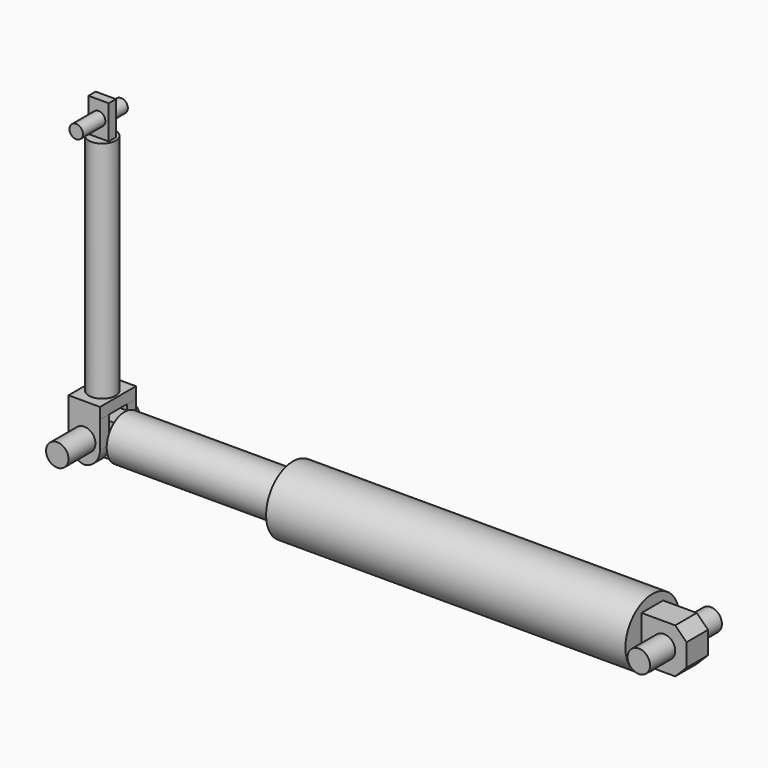
from build123d import *

# Parameters (mm, degrees)
F0_R         = 10
F1_DEPTH     = 75
F2_R         = 15
F2_R_2       = 10
F3_DEPTH     = 150
F4_R         = 15
F5_DEPTH     = 10
F6_W         = 12
F6_H         = 20
F7_DEPTH     = 20
F8_R         = 5
F9_DEPTH     = 21.001
F10_SIZE     = 5
F11_W        = 10
F11_H        = 15
F12_DEPTH    = 20
F13_R        = 5
F14_DEPTH    = 20.001
F15_R        = 5
F16_DEPTH    = 20
F17_W        = 14
F17_H        = 5
F18_DEPTH    = 10
F19_W        = 14.032341361
F19_H        = 20.0174024701
F20_DEPTH    = 5
F21_R        = 5
F22_DEPTH    = 20
F24_T1_DEPTH = 45
F24_T3_DEPTH = 45
F25_R        = 6
F26_DEPTH    = 100
F27_W        = 9
F27_H        = 4
F28_DEPTH    = 15
F29_R        = 3
F30_DEPTH    = 12.5
F32_T1_DEPTH = 50


# Not quite as in the source:
# - a fillet or chamfer that OpenCascade refuses, or shapes differently, is made with other operations: its cross-section is extruded or revolved along the edge and cut away or added


with BuildPart() as f1:
    # F0 (on Right) → F1 (new body, symmetric)
    with BuildSketch(Plane.YZ):
        Circle(F0_R)
    extrude(amount=F1_DEPTH, both=True)

    # F11 (on face) → F12 (join)
    with BuildSketch(Plane(origin=(-75, 0, 0), x_dir=(0, -1, 0), z_dir=(-1, 0, 0))):
        Rectangle(F11_W, F11_H)
    extrude(amount=F12_DEPTH)

    # F13 (on face) → F14 (cut, through all)
    with BuildSketch(Plane.XZ.offset(5)):
        with Locations((-85, 0)):
            Circle(F13_R)
    extrude(amount=-F14_DEPTH, mode=Mode.SUBTRACT)

    # F32: fillet of radius 8 on 2 edges, made by hand

    # F32_s2 → F32_t1 (cut)
    with BuildSketch(Plane.XZ.offset(-25)):
        with BuildLine():
            ThreePointArc((-87, 7.5), (-92.6568542495, 5.1568542495), (-95, -0.5))
            Line((-95, -0.5), (-95, 7.5))
            Line((-95, 7.5), (-87, 7.5))
        make_face()
        with BuildLine():
            ThreePointArc((-87, -7.5), (-92.6568542495, -5.1568542495), (-95, 0.5))
            Line((-95, 0.5), (-95, -7.5))
            Line((-95, -7.5), (-87, -7.5))
        make_face()
    extrude(amount=F32_T1_DEPTH, mode=Mode.SUBTRACT)


with BuildPart() as f3:
    # F2 (on Right) → F3 (new body)
    with BuildSketch(Plane.YZ):
        Circle(F2_R)
        Circle(F2_R_2, mode=Mode.SUBTRACT)
    extrude(amount=F3_DEPTH)

    # F4 (on face) → F5 (join)
    with BuildSketch(Plane.YZ.offset(150)):
        Circle(F4_R)
    extrude(amount=F5_DEPTH)

    # F6 (on face) → F7 (join)
    with BuildSketch(Plane.YZ.offset(160)):
        Rectangle(F6_W, F6_H)
    extrude(amount=F7_DEPTH)

    # F8 (on face) → F9 (cut, through all)
    with BuildSketch(Plane.XZ.offset(6)):
        with Locations((170, 0)):
            Circle(F8_R)
    extrude(amount=-F9_DEPTH, mode=Mode.SUBTRACT)

    # F10
    f10_edges = [f3.edges().sort_by_distance(p)[0] for p in [
        (180, 0, 10),
        (180, 0, -10),
    ]]
    chamfer(f10_edges, length=F10_SIZE)


with BuildPart() as f16:
    # F15 (on Front) → F16 (new body, symmetric)
    with BuildSketch(Plane.XZ):
        with Locations((170, 0)):
            Circle(F15_R)
    extrude(amount=F16_DEPTH, both=True)


with BuildPart() as f18:
    # F17 (on Top) → F18 (new body, symmetric)
    with BuildSketch(Plane.XY):
        with Locations((-85, 7.5)):
            Rectangle(F17_W, F17_H)
    extrude(amount=F18_DEPTH, both=True)



with BuildPart() as f18b:
    # F17 (on Top) → F18, piece 2 (new body, symmetric)
    with BuildSketch(Plane.XY):
        with Locations((-85, -7.5)):
            Rectangle(F17_W, F17_H)
    extrude(amount=F18_DEPTH, both=True)


with BuildPart() as f18_1:
    add(f18.part)

    add(f18b.part)  # F20 merges F18b
    # F19 (on face) → F20 (join)
    with BuildSketch(Plane.XY.offset(10)):
        with Locations((-84.9838293195, 0.0087012351)):
            Rectangle(F19_W, F19_H)
    extrude(amount=F20_DEPTH)


with BuildPart() as f22:
    # F21 (on face) → F22 (new body, symmetric)
    with BuildSketch(Plane.XZ.offset(5)):
        with Locations((-85, 0)):
            Circle(F21_R)
    extrude(amount=F22_DEPTH, both=True)


with BuildPart() as f18_2:
    add(f18_1.part)

    # F23: cut F22
    add(f22.part, mode=Mode.SUBTRACT)

    # F24: fillet of radius 8 on 4 edges, made by hand

    # F24_s2 → F24_t1 (cut)
    with BuildSketch(Plane.XZ.offset(-30)):
        with BuildLine():
            ThreePointArc((-92, -2), (-89.6568542495, -7.6568542495), (-84, -10))
            Line((-84, -10), (-92, -10))
            Line((-92, -10), (-92, -2))
        make_face()
        with BuildLine():
            ThreePointArc((-86, -10), (-80.3431457505, -7.6568542495), (-78, -2))
            Line((-78, -2), (-78, -10))
            Line((-78, -10), (-86, -10))
        make_face()
    extrude(amount=F24_T1_DEPTH, mode=Mode.SUBTRACT)

    # F24_s4 → F24_t3 (cut)
    with BuildSketch(Plane.XZ.offset(-15)):
        with BuildLine():
            ThreePointArc((-86, -10), (-80.3431457505, -7.6568542495), (-78, -2))
            Line((-78, -2), (-78, -10))
            Line((-78, -10), (-86, -10))
        make_face()
        with BuildLine():
            ThreePointArc((-84, -10), (-89.6568542495, -7.6568542495), (-92, -2))
            Line((-92, -2), (-92, -10))
            Line((-92, -10), (-84, -10))
        make_face()
    extrude(amount=F24_T3_DEPTH, mode=Mode.SUBTRACT)

    # F25 (on face) → F26 (join)
    with BuildSketch(Plane.XY.offset(15)):
        with Locations((-84.9899289471, 0)):
            Circle(F25_R)
    extrude(amount=F26_DEPTH)

    # F27 (on face) → F28 (join)
    with BuildSketch(Plane.XY.offset(115)):
        with Locations((-84.9899289471, 0)):
            Rectangle(F27_W, F27_H)
    extrude(amount=F28_DEPTH)


with BuildPart() as f30:
    # F29 (on face) → F30 (new body, symmetric)
    with BuildSketch(Plane.XZ.offset(2)):
        with Locations((-84.9899289471, 122.5)):
            Circle(F29_R)
    extrude(amount=F30_DEPTH, both=True)


with BuildPart() as f18_3:
    add(f18_2.part)

    # F31: cut F30
    add(f30.part, mode=Mode.SUBTRACT)


solid = Compound([f1.part, f3.part, f16.part, f22.part, f30.part, f18_3.part])
